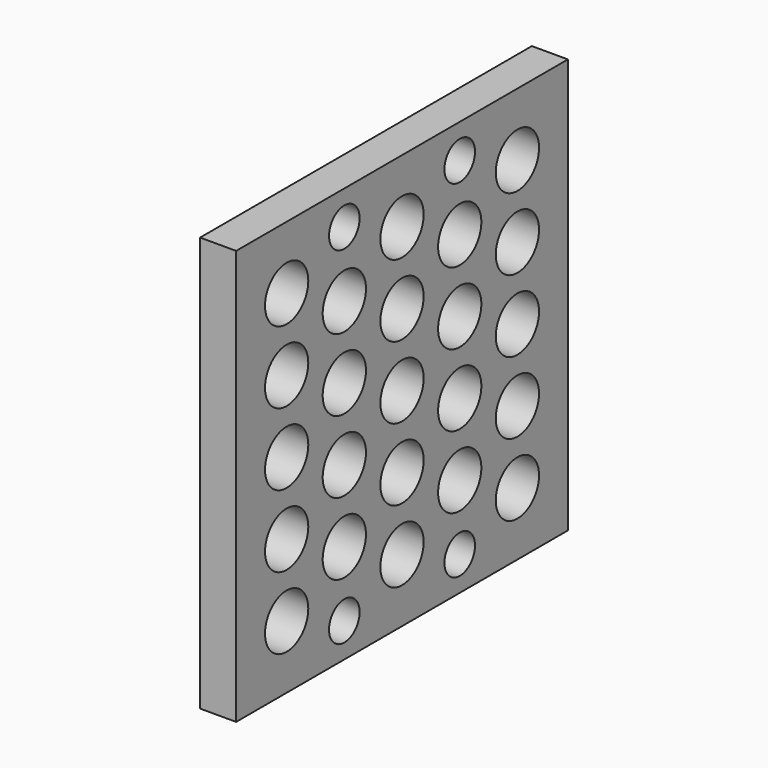
from build123d import *

# Parameters (mm, degrees)
F0_R     = 0.75
F0_R_2   = 0.53
F1_DEPTH = 1


# Not quite as in the source:
# - a feature names something its author has since deleted; it is built from what else it names


with BuildPart() as f1:
    # F0 (on Right) → F1 (new body)
    with BuildSketch(Plane.YZ):
        Polygon((8.384144865, 0), (0, 0), (0, -11.5), (11.5, -11.5), (11.5, 0), (10.384144865, 0), align=None)
        with Locations((1.7500000088, -9.75)):
            Circle(F0_R, mode=Mode.SUBTRACT)
        with Locations((1.75, -7.75)):
            Circle(F0_R, mode=Mode.SUBTRACT)
        with Locations((3.7499851588, -10.5567658602)):
            Circle(F0_R_2, mode=Mode.SUBTRACT)
        with Locations((5.7499653617, -9.750009894)):
            Circle(F0_R, mode=Mode.SUBTRACT)
        with Locations((3.7499885936, -8.7499999912)):
            Circle(F0_R, mode=Mode.SUBTRACT)
        with Locations((3.7499923957, -6.75)):
            Circle(F0_R, mode=Mode.SUBTRACT)
        with Locations((5.7499752647, -7.7500098941)):
            Circle(F0_R, mode=Mode.SUBTRACT)
        with Locations((1.75, -5.75)):
            Circle(F0_R, mode=Mode.SUBTRACT)
        with Locations((1.75, -3.75)):
            Circle(F0_R, mode=Mode.SUBTRACT)
        with Locations((1.75, -1.75)):
            Circle(F0_R, mode=Mode.SUBTRACT)
        with Locations((3.7499961979, -4.75)):
            Circle(F0_R, mode=Mode.SUBTRACT)
        with Locations((5.7499851588, -5.7500098941)):
            Circle(F0_R, mode=Mode.SUBTRACT)
        with Locations((5.7499950529, -3.7500098941)):
            Circle(F0_R, mode=Mode.SUBTRACT)
        with Locations((3.75, -2.75)):
            Circle(F0_R, mode=Mode.SUBTRACT)
        with Locations((3.75, -0.94325)):
            Circle(F0_R_2, mode=Mode.SUBTRACT)
        with Locations((7.749955461, -10.5567658602)):
            Circle(F0_R_2, mode=Mode.SUBTRACT)
        with Locations((7.7499520262, -8.7500197836)):
            Circle(F0_R, mode=Mode.SUBTRACT)
        with Locations((7.7499680167, -6.7500197925)):
            Circle(F0_R, mode=Mode.SUBTRACT)
        with Locations((9.7499307145, -9.750039585)):
            Circle(F0_R, mode=Mode.SUBTRACT)
        with Locations((9.749950516, -7.7500395851)):
            Circle(F0_R, mode=Mode.SUBTRACT)
        with Locations((7.7499840072, -4.7500197926)):
            Circle(F0_R, mode=Mode.SUBTRACT)
        with Locations((5.750004947, -1.7500098941)):
            Circle(F0_R, mode=Mode.SUBTRACT)
        with Locations((7.7499999977, -2.7500197927)):
            Circle(F0_R, mode=Mode.SUBTRACT)
        with Locations((7.7499999977, -0.9432697927)):
            Circle(F0_R_2, mode=Mode.SUBTRACT)
        with Locations((9.7499703087, -5.7500395852)):
            Circle(F0_R, mode=Mode.SUBTRACT)
        with Locations((9.7499901013, -3.7500395853)):
            Circle(F0_R, mode=Mode.SUBTRACT)
        with Locations((9.750009894, -1.7500395854)):
            Circle(F0_R, mode=Mode.SUBTRACT)
    extrude(amount=F1_DEPTH)


solid = f1.part
